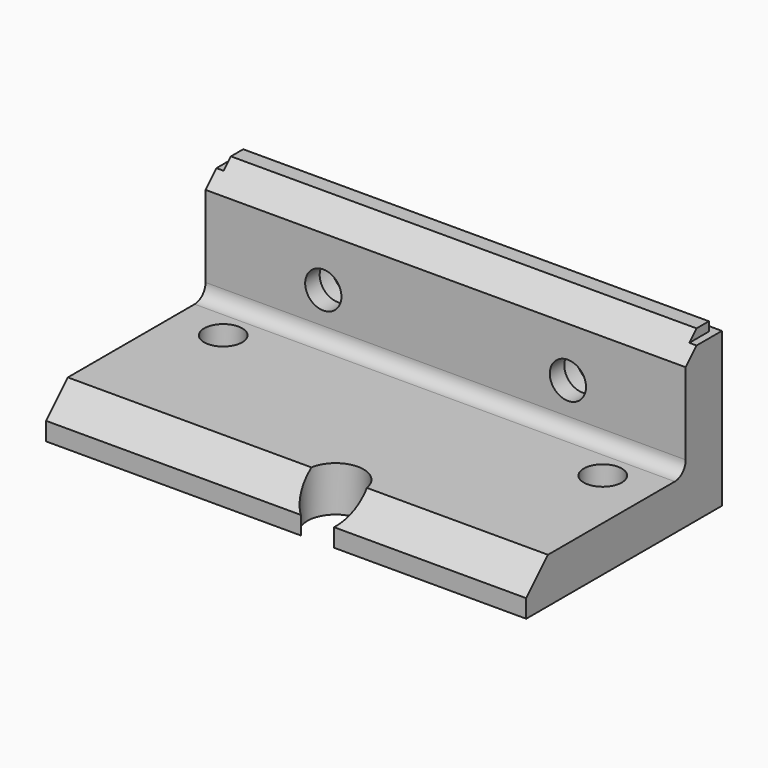
from build123d import *

# Parameters (mm, degrees)
F0_R           = 3.1
F0_W           = 53
F0_H           = 5
F0_R_2         = 2.1
F1_DEPTH       = 5
F2_DEPTH       = 2.1
F3_DEPTH       = 18
F4_W           = 0.8
F4_H           = 1
F4_W_2         = 51.4
F5_DEPTH       = 0.8
F6_DEPTH       = 25
F7_D           = 4
F7_CBORE_D     = 6.6
F7_CBORE_DEPTH = 3
F8_SIZE        = 2.5
F9_R           = 1.5
F10_SIZE       = 3


with BuildPart() as f1:
    # F0 (on Top) → F1 (new body)
    with BuildSketch(Plane.XY):
        with BuildLine():
            Line((26.5, -5), (-26.5, -5))
            Line((-26.5, -5), (-26.5, -27))
            Line((-26.5, -27), (1.616969722, -27))
            ThreePointArc((1.616969722, -27), (2.0486424192, -21.7348242496), (6.55, -24.5))
            ThreePointArc((6.55, -24.5), (6.2151757504, -25.9013575808), (5.283030278, -27))
            Line((5.283030278, -27), (26.5, -27))
            Line((26.5, -27), (26.5, -5))
        make_face()
        with Locations((-20.95, -9.5)):
            Circle(F0_R, mode=Mode.SUBTRACT)
        with Locations((20.95, -9.5)):
            Circle(F0_R, mode=Mode.SUBTRACT)
        with Locations((0, -2.5)):
            Rectangle(F0_W, F0_H)
        with Locations((-20.95, -9.5)):
            Circle(F0_R)
        with Locations((-20.95, -9.5)):
            Circle(F0_R_2, mode=Mode.SUBTRACT)
        with Locations((20.95, -9.5)):
            Circle(F0_R)
        with Locations((20.95, -9.5)):
            Circle(F0_R_2, mode=Mode.SUBTRACT)
    extrude(amount=F1_DEPTH)

    # F0 (on Top) → F2 (cut)
    with BuildSketch(Plane.XY):
        with Locations((20.95, -9.5)):
            Circle(F0_R)
        with Locations((20.95, -9.5)):
            Circle(F0_R_2, mode=Mode.SUBTRACT)
        with Locations((-20.95, -9.5)):
            Circle(F0_R)
        with Locations((-20.95, -9.5)):
            Circle(F0_R_2, mode=Mode.SUBTRACT)
    extrude(amount=F2_DEPTH, mode=Mode.SUBTRACT)

    # F0 (on Top) → F3 (join)
    with BuildSketch(Plane.XY):
        with Locations((0, -2.5)):
            Rectangle(F0_W, F0_H)
    extrude(amount=F3_DEPTH)

    # F4 (on face) → F5 (cut)
    with BuildSketch(Plane(origin=(0, 0, 0), x_dir=(-1, 0, 0), z_dir=(0, 1, 0))):
        with Locations((-26.1, 17.5)):
            Rectangle(F4_W, F4_H)
        with Locations((0, 17.5)):
            Rectangle(F4_W_2, F4_H)
        with Locations((26.1, 17.5)):
            Rectangle(F4_W, F4_H)
    extrude(amount=-F5_DEPTH, mode=Mode.SUBTRACT)

    # F4 (on face) → F6 (cut)
    with BuildSketch(Plane(origin=(0, 0, 0), x_dir=(-1, 0, 0), z_dir=(0, 1, 0))):
        with Locations((-26.1, 17.5)):
            Rectangle(F4_W, F4_H)
        with Locations((26.1, 17.5)):
            Rectangle(F4_W, F4_H)
    extrude(amount=-F6_DEPTH, mode=Mode.SUBTRACT)

    # F7 (through all)
    with Locations(Plane(origin=(0, 0, 0), x_dir=(-1, 0, 0), z_dir=(0, 1, 0))):
        with Locations((13.5, 10), (-13.5, 10)):
            CounterBoreHole(F7_D / 2, F7_CBORE_D / 2, F7_CBORE_DEPTH)

    # F8
    f8_edges = [f1.edges().sort_by_distance(p)[0] for p in [
        (0, -5, 18),
    ]]
    chamfer(f8_edges, length=F8_SIZE)

    # F9
    f9_edges = [f1.edges().sort_by_distance(p)[0] for p in [
        (0, -5, 5),
    ]]
    fillet(f9_edges, radius=F9_R)

    # F10
    f10_edges = [f1.edges().sort_by_distance(p)[0] for p in [
        (15.891515, -27, 5),
        (-12.441515, -27, 5),
    ]]
    chamfer(f10_edges, length=F10_SIZE)


solid = f1.part
